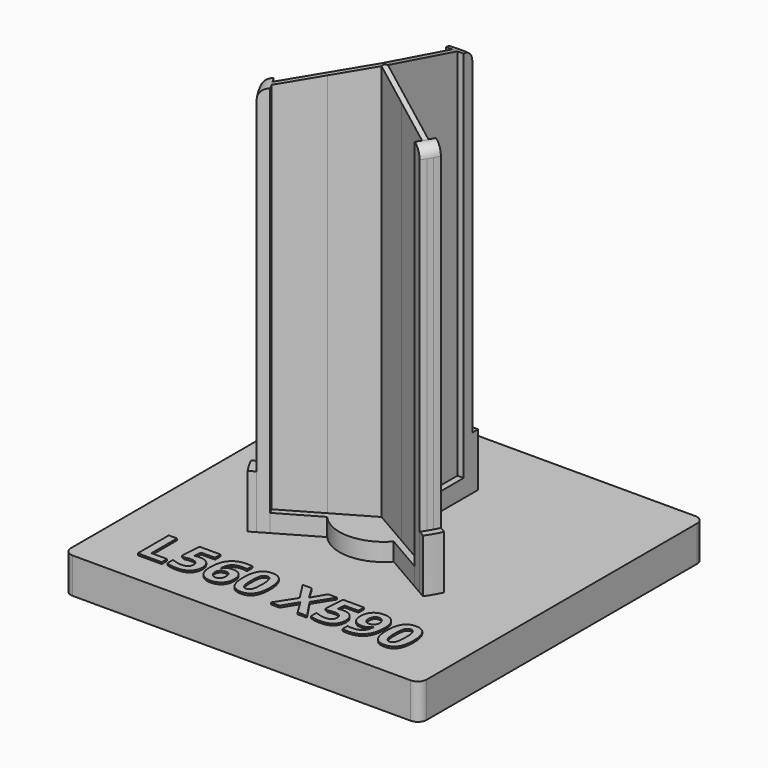
from build123d import *

# Parameters (mm, degrees)
F0_R         = 3.5
F0_R_2       = 1.75
F1_DEPTH     = 10
F2_DEPTH     = 220
F3_DEPTH     = 235
F4_T4_DEPTH  = 293.7329049929
F4_T9_DEPTH  = 293.7329049929
F4_T14_DEPTH = 293.7329049929
F5_T2_ANGLE  = 40.9393595263
F5_T4_ANGLE  = 40.9393595263
F5_T6_ANGLE  = 40.9393595263
F6_DEPTH     = 3
F7_DEPTH     = 30
F8_W         = 200
F8_H         = 200
F9_DEPTH     = 20
F10_R        = 5
F0_TEXT_SIZE = 30.5555555556
F11_DEPTH    = 1


# Not quite as in the source:
# - a fillet or chamfer that OpenCascade refuses, or shapes differently, is made with other operations: its cross-section is extruded or revolved along the edge and cut away or added
# - a feature names something its author has since deleted; it is built from what else it names
# - Text() gives the source's letters only with a copy of the font that has no kerning and outlines rounded to 1/6400 em; it was checked with that copy


with BuildPart() as f1:
    # F0 (on Top) → F1 (new body)
    with BuildSketch(Plane.XY):
        with BuildLine():
            ThreePointArc((25, 0), (19.364916731, 15.8113883008), (5, 24.4948974278))
            ThreePointArc((5, 24.4948974278), (3.2581304855, 24.7867824806), (1.5, 24.9549594269))
            Line((1.5, 24.9549594269), (1.5, 0.8660254038))
            Line((1.5, 0.8660254038), (22.3616288141, -11.1784416078))
            ThreePointArc((22.3616288141, -11.1784416078), (23.095048549, -9.571767471), (23.7132034356, -7.917321695))
            ThreePointArc((23.7132034356, -7.917321695), (24.6762039817, -4.0106055721), (25, 0))
        make_face()
        with Locations((11.9308144071, 6.8882589096)):
            Circle(F0_R, mode=Mode.SUBTRACT)
        with BuildLine():
            Line((5, 24.4948974278), (5, 49.7493718553))
            Line((5, 49.7493718553), (1.5, 49.7493718553))
            Line((1.5, 49.7493718553), (1.5, 24.9549594269))
            ThreePointArc((1.5, 24.9549594269), (3.2581304855, 24.7867824806), (5, 24.4948974278))
        make_face()
        with BuildLine():
            Line((43.834219849, -23.575647822), (45.584219849, -20.5445589087))
            Line((45.584219849, -20.5445589087), (23.7132034356, -7.917321695))
            ThreePointArc((23.7132034356, -7.917321695), (23.095048549, -9.571767471), (22.3616288141, -11.1784416078))
            Line((22.3616288141, -11.1784416078), (43.834219849, -23.575647822))
        make_face()
        with Locations((11.9308144071, 6.8882589096)):
            Circle(F0_R)
        with Locations((11.9308144071, 6.8882589096)):
            Circle(F0_R_2, mode=Mode.SUBTRACT)
        with Locations((11.9308144071, 6.8882589096)):
            Circle(F0_R_2)
    extrude(amount=F1_DEPTH)



with BuildPart() as f1b:
    # F0 (on Top) → F1, piece 2 (new body)
    with BuildSketch(Plane.XY):
        with BuildLine():
            Line((-1.5, 49.7493718553), (-5, 49.7493718553))
            Line((-5, 49.7493718553), (-5, 24.4948974278))
            ThreePointArc((-5, 24.4948974278), (-3.2581304855, 24.7867824806), (-1.5, 24.9549594269))
            Line((-1.5, 24.9549594269), (-1.5, 49.7493718553))
        make_face()
        with BuildLine():
            Line((-23.7132034356, -7.917321695), (-45.584219849, -20.5445589087))
            Line((-45.584219849, -20.5445589087), (-43.834219849, -23.575647822))
            Line((-43.834219849, -23.575647822), (-22.3616288141, -11.1784416078))
            ThreePointArc((-22.3616288141, -11.1784416078), (-23.095048549, -9.571767471), (-23.7132034356, -7.917321695))
        make_face()
        with BuildLine():
            ThreePointArc((-1.5, 24.9549594269), (-3.2581304855, 24.7867824806), (-5, 24.4948974278))
            ThreePointArc((-5, 24.4948974278), (-21.6506350946, 12.5), (-23.7132034356, -7.917321695))
            ThreePointArc((-23.7132034356, -7.917321695), (-23.095048549, -9.571767471), (-22.3616288141, -11.1784416078))
            Line((-22.3616288141, -11.1784416078), (-1.5, 0.8660254038))
            Line((-1.5, 0.8660254038), (-1.5, 24.9549594269))
        make_face()
        with Locations((-11.9308144071, 6.8882589096)):
            Circle(F0_R, mode=Mode.SUBTRACT)
        with Locations((-11.9308144071, 6.8882589096)):
            Circle(F0_R)
        with Locations((-11.9308144071, 6.8882589096)):
            Circle(F0_R_2, mode=Mode.SUBTRACT)
        with Locations((-11.9308144071, 6.8882589096)):
            Circle(F0_R_2)
    extrude(amount=F1_DEPTH)


with BuildPart() as f1c:
    # F0 (on Top) → F1, piece 3 (new body)
    with BuildSketch(Plane.XY):
        with BuildLine():
            ThreePointArc((-18.7132034356, -16.5775757328), (0, -25), (18.7132034356, -16.5775757328))
            ThreePointArc((18.7132034356, -16.5775757328), (19.8369180635, -15.2150150096), (20.8616288141, -13.7765178191))
            Line((20.8616288141, -13.7765178191), (0, -1.7320508076))
            Line((0, -1.7320508076), (-20.8616288141, -13.7765178191))
            ThreePointArc((-20.8616288141, -13.7765178191), (-19.8369180635, -15.2150150096), (-18.7132034356, -16.5775757328))
        make_face()
        with Locations((0, -13.7765178191)):
            Circle(F0_R, mode=Mode.SUBTRACT)
        with BuildLine():
            Line((18.7132034356, -16.5775757328), (40.584219849, -29.2048129466))
            Line((40.584219849, -29.2048129466), (42.334219849, -26.1737240333))
            Line((42.334219849, -26.1737240333), (20.8616288141, -13.7765178191))
            ThreePointArc((20.8616288141, -13.7765178191), (19.8369180635, -15.2150150096), (18.7132034356, -16.5775757328))
        make_face()
        with BuildLine():
            Line((-42.334219849, -26.1737240333), (-40.584219849, -29.2048129466))
            Line((-40.584219849, -29.2048129466), (-18.7132034356, -16.5775757328))
            ThreePointArc((-18.7132034356, -16.5775757328), (-19.8369180635, -15.2150150096), (-20.8616288141, -13.7765178191))
            Line((-20.8616288141, -13.7765178191), (-42.334219849, -26.1737240333))
        make_face()
        with Locations((0, -13.7765178191)):
            Circle(F0_R)
        with Locations((0, -13.7765178191)):
            Circle(F0_R_2, mode=Mode.SUBTRACT)
        with Locations((0, -13.7765178191)):
            Circle(F0_R_2)
    extrude(amount=F1_DEPTH)


with BuildPart() as f1_1:
    add(f1.part)

    add(f1b.part)  # F2 merges F1b

    add(f1c.part)  # F2 merges F1c
    # F0 (on Top) → F2 (join)
    with BuildSketch(Plane.XY):
        with BuildLine():
            Line((5, 49.7493718553), (5, 55.7763390695))
            ThreePointArc((5, 55.7763390695), (3.2515934535, 55.9055197634), (1.5, 55.9799071096))
            Line((1.5, 55.9799071096), (1.5, 49.7493718553))
            Line((1.5, 49.7493718553), (5, 49.7493718553))
        make_face()
        with BuildLine():
            ThreePointArc((-1.5, 55.9799071096), (-3.2515934535, 55.9055197634), (-5, 55.7763390695))
            Line((-5, 55.7763390695), (-5, 49.7493718553))
            Line((-5, 49.7493718553), (-1.5, 49.7493718553))
            Line((-1.5, 49.7493718553), (-1.5, 55.9799071096))
        make_face()
        with BuildLine():
            ThreePointArc((-47.7300216584, -29.2889916605), (-46.7898036001, -30.7687224152), (-45.8037265643, -32.2182965537))
            Line((-45.8037265643, -32.2182965537), (-40.584219849, -29.2048129466))
            Line((-40.584219849, -29.2048129466), (-42.334219849, -26.1737240333))
            Line((-42.334219849, -26.1737240333), (-47.7300216584, -29.2889916605))
        make_face()
        with BuildLine():
            Line((-45.584219849, -20.5445589087), (-50.8037265643, -23.5580425158))
            ThreePointArc((-50.8037265643, -23.5580425158), (-50.0413970536, -25.1367973482), (-49.2300216584, -26.6909154491))
            Line((-49.2300216584, -26.6909154491), (-43.834219849, -23.575647822))
            Line((-43.834219849, -23.575647822), (-45.584219849, -20.5445589087))
        make_face()
        with BuildLine():
            Line((40.584219849, -29.2048129466), (45.8037265643, -32.2182965537))
            ThreePointArc((45.8037265643, -32.2182965537), (46.7898036001, -30.7687224152), (47.7300216584, -29.2889916605))
            Line((47.7300216584, -29.2889916605), (42.334219849, -26.1737240333))
            Line((42.334219849, -26.1737240333), (40.584219849, -29.2048129466))
        make_face()
        with BuildLine():
            ThreePointArc((49.2300216584, -26.6909154491), (50.0413970536, -25.1367973482), (50.8037265643, -23.5580425158))
            Line((50.8037265643, -23.5580425158), (45.584219849, -20.5445589087))
            Line((45.584219849, -20.5445589087), (43.834219849, -23.575647822))
            Line((43.834219849, -23.575647822), (49.2300216584, -26.6909154491))
        make_face()
        with BuildLine():
            Line((-43.834219849, -23.575647822), (-49.2300216584, -26.6909154491))
            ThreePointArc((-49.2300216584, -26.6909154491), (-48.4974226119, -28), (-47.7300216584, -29.2889916605))
            Line((-47.7300216584, -29.2889916605), (-42.334219849, -26.1737240333))
            Line((-42.334219849, -26.1737240333), (-43.834219849, -23.575647822))
        make_face()
        with BuildLine():
            ThreePointArc((47.7300216584, -29.2889916605), (48.4974226119, -28), (49.2300216584, -26.6909154491))
            Line((49.2300216584, -26.6909154491), (43.834219849, -23.575647822))
            Line((43.834219849, -23.575647822), (42.334219849, -26.1737240333))
            Line((42.334219849, -26.1737240333), (47.7300216584, -29.2889916605))
        make_face()
        with BuildLine():
            Line((1.5, 49.7493718553), (1.5, 55.9799071096))
            ThreePointArc((1.5, 55.9799071096), (0, 56), (-1.5, 55.9799071096))
            Line((-1.5, 55.9799071096), (-1.5, 49.7493718553))
            Line((-1.5, 49.7493718553), (1.5, 49.7493718553))
        make_face()
    extrude(amount=F2_DEPTH)

    # F0 (on Top) → F3 (join)
    with BuildSketch(Plane.XY):
        with BuildLine():
            Line((1.5, 0.8660254038), (1.5, 24.9549594269))
            ThreePointArc((1.5, 24.9549594269), (0, 25), (-1.5, 24.9549594269))
            Line((-1.5, 24.9549594269), (-1.5, 0.8660254038))
            Line((-1.5, 0.8660254038), (-22.3616288141, -11.1784416078))
            ThreePointArc((-22.3616288141, -11.1784416078), (-21.6506350946, -12.5), (-20.8616288141, -13.7765178191))
            Line((-20.8616288141, -13.7765178191), (0, -1.7320508076))
            Line((0, -1.7320508076), (20.8616288141, -13.7765178191))
            ThreePointArc((20.8616288141, -13.7765178191), (21.6506350946, -12.5), (22.3616288141, -11.1784416078))
            Line((22.3616288141, -11.1784416078), (1.5, 0.8660254038))
        make_face()
        with BuildLine():
            Line((1.5, 24.9549594269), (1.5, 49.7493718553))
            Line((1.5, 49.7493718553), (-1.5, 49.7493718553))
            Line((-1.5, 49.7493718553), (-1.5, 24.9549594269))
            ThreePointArc((-1.5, 24.9549594269), (0, 25), (1.5, 24.9549594269))
        make_face()
        with BuildLine():
            Line((-22.3616288141, -11.1784416078), (-43.834219849, -23.575647822))
            Line((-43.834219849, -23.575647822), (-42.334219849, -26.1737240333))
            Line((-42.334219849, -26.1737240333), (-20.8616288141, -13.7765178191))
            ThreePointArc((-20.8616288141, -13.7765178191), (-21.6506350946, -12.5), (-22.3616288141, -11.1784416078))
        make_face()
        with BuildLine():
            Line((42.334219849, -26.1737240333), (43.834219849, -23.575647822))
            Line((43.834219849, -23.575647822), (22.3616288141, -11.1784416078))
            ThreePointArc((22.3616288141, -11.1784416078), (21.6506350946, -12.5), (20.8616288141, -13.7765178191))
            Line((20.8616288141, -13.7765178191), (42.334219849, -26.1737240333))
        make_face()
    extrude(amount=F3_DEPTH)

    # F4: chamfer of 15 x 55.9807621135 on 3 edges, made by hand


with BuildPart() as f4_tool2:
    # F4_s3 → F4_t4 (new body)
    with BuildSketch(Plane(origin=(-73.4332262482, -127.1900788256, 0), x_dir=(0, 0, 1), z_dir=(0.5, 0.8660254038, 0))):
        Polygon((220, 49.7493718553), (235, -6.2313902582), (235, 49.7493718553), align=None)
    extrude(amount=F4_T4_DEPTH)

    split(bisect_by=Plane.XY.offset(220), keep=Keep.TOP)


with BuildPart() as f1_2:
    add(f1_1.part)

    # F4_t1: cut F4_tool2
    add(f4_tool2.part, mode=Mode.SUBTRACT)


with BuildPart() as f4_tool7:
    # F4_s8 → F4_t9 (new body)
    with BuildSketch(Plane(origin=(-73.4332262482, 127.1900788256, 0), x_dir=(0, 0, 1), z_dir=(0.5, -0.8660254038, 0))):
        Polygon((235, -6.2313902582), (220, 49.7493718553), (235, 49.7493718553), align=None)
    extrude(amount=F4_T9_DEPTH)

    split(bisect_by=Plane.XY.offset(220), keep=Keep.TOP)


with BuildPart() as f1_3:
    add(f1_2.part)

    # F4_t6: cut F4_tool7
    add(f4_tool7.part, mode=Mode.SUBTRACT)


with BuildPart() as f4_tool12:
    # F4_s13 → F4_t14 (new body)
    with BuildSketch(Plane.YZ.offset(146.8664524965)):
        Polygon((-6.2313902582, 235), (49.7493718553, 220), (49.7493718553, 235), align=None)
    extrude(amount=-F4_T14_DEPTH)

    split(bisect_by=Plane.XY.offset(220), keep=Keep.TOP)


with BuildPart() as f1_4:
    add(f1_3.part)

    # F4_t11: cut F4_tool12
    add(f4_tool12.part, mode=Mode.SUBTRACT)

    # F5: fillet of radius 6 on 3 edges, made by hand

    # F5_s1 → F5_t2 (revolve, cut)
    with BuildSketch(Plane(origin=(0, 0, 0), x_dir=(0, 0, 1), z_dir=(-0.7712878704, -0.6364864656, 0))):
        with BuildLine():
            ThreePointArc((220, -50), (218.2426406871, -54.2426406871), (214, -56))
            Line((214, -56), (220, -56))
            Line((220, -56), (220, -50))
        make_face()
    revolve(axis=Axis((0, 0, 220), (0, 0, 1)), revolution_arc=F5_T2_ANGLE, mode=Mode.SUBTRACT)

    # F5_s3 → F5_t4 (revolve, cut)
    with BuildSketch(Plane(origin=(0, 0, 0), x_dir=(0, 0, 1), z_dir=(0.9368573836, -0.3497116566, 0))):
        with BuildLine():
            ThreePointArc((214, -56), (218.2426406871, -54.2426406871), (220, -50))
            Line((220, -50), (220, -56))
            Line((220, -56), (214, -56))
        make_face()
    revolve(axis=Axis((0, 0, 220), (0, 0, 1)), revolution_arc=F5_T4_ANGLE, mode=Mode.SUBTRACT)

    # F5_s5 → F5_t6 (revolve, cut)
    with BuildSketch(Plane(origin=(0, 0, 0), x_dir=(0, 0, 1), z_dir=(-0.1655695132, 0.9861981222, 0))):
        with BuildLine():
            ThreePointArc((214, -56), (218.2426406871, -54.2426406871), (220, -50))
            Line((220, -50), (220, -56))
            Line((220, -56), (214, -56))
        make_face()
    revolve(axis=Axis((0, 0, 220), (0, 0, 1)), revolution_arc=F5_T6_ANGLE, mode=Mode.SUBTRACT)

    # F0 (on Top) → F6 (join)
    with BuildSketch(Plane.XY):
        with Locations((-11.9308144071, 6.8882589096)):
            Circle(F0_R)
        with Locations((-11.9308144071, 6.8882589096)):
            Circle(F0_R_2, mode=Mode.SUBTRACT)
        with Locations((0, -13.7765178191)):
            Circle(F0_R)
        with Locations((0, -13.7765178191)):
            Circle(F0_R_2, mode=Mode.SUBTRACT)
        with Locations((11.9308144071, 6.8882589096)):
            Circle(F0_R)
        with Locations((11.9308144071, 6.8882589096)):
            Circle(F0_R_2, mode=Mode.SUBTRACT)
    extrude(amount=F6_DEPTH)

    # F0 (on Top) → F7 (join)
    with BuildSketch(Plane.XY):
        with BuildLine():
            Line((-50.8037265643, -23.5580425158), (-54.280787943, -25.5655248388))
            ThreePointArc((-54.280787943, -25.5655248388), (-51.9615242271, -30), (-49.280787943, -34.2257788767))
            Line((-49.280787943, -34.2257788767), (-45.8037265643, -32.2182965537))
            ThreePointArc((-45.8037265643, -32.2182965537), (-46.7898036001, -30.7687224152), (-47.7300216584, -29.2889916605))
            ThreePointArc((-47.7300216584, -29.2889916605), (-48.4974226119, -28), (-49.2300216584, -26.6909154491))
            ThreePointArc((-49.2300216584, -26.6909154491), (-50.0413970536, -25.1367973482), (-50.8037265643, -23.5580425158))
        make_face()
        with BuildLine():
            ThreePointArc((49.280787943, -34.2257788767), (51.9615242271, -30), (54.280787943, -25.5655248388))
            Line((54.280787943, -25.5655248388), (50.8037265643, -23.5580425158))
            ThreePointArc((50.8037265643, -23.5580425158), (50.0413970536, -25.1367973482), (49.2300216584, -26.6909154491))
            ThreePointArc((49.2300216584, -26.6909154491), (48.4974226119, -28), (47.7300216584, -29.2889916605))
            ThreePointArc((47.7300216584, -29.2889916605), (46.7898036001, -30.7687224152), (45.8037265643, -32.2182965537))
            Line((45.8037265643, -32.2182965537), (49.280787943, -34.2257788767))
        make_face()
        with BuildLine():
            Line((5, 55.7763390695), (5, 59.7913037155))
            ThreePointArc((5, 59.7913037155), (0, 60), (-5, 59.7913037155))
            Line((-5, 59.7913037155), (-5, 55.7763390695))
            ThreePointArc((-5, 55.7763390695), (-3.2515934535, 55.9055197634), (-1.5, 55.9799071096))
            ThreePointArc((-1.5, 55.9799071096), (0, 56), (1.5, 55.9799071096))
            ThreePointArc((1.5, 55.9799071096), (3.2515934535, 55.9055197634), (5, 55.7763390695))
        make_face()
    extrude(amount=F7_DEPTH)

    # F8 (on Top) → F9 (join)
    with BuildSketch(Plane.XY):
        Rectangle(F8_W, F8_H)
    extrude(amount=-F9_DEPTH)

    # F10
    f10_edges = [f1_4.edges().sort_by_distance(p)[0] for p in [
        (-100, -100, -10),
        (100, -100, -10),
        (100, 100, -10),
        (-100, 100, -10),
    ]]
    fillet(f10_edges, radius=F10_R)

    # F0 (on Top) → F11 (join)
    with BuildSketch(Plane.XY):
        with Locations((-75.560546875, -82)):
            Text('L560 X590', F0_TEXT_SIZE, font='Open Sans', font_style=FontStyle.BOLD, text_align=(TextAlign.LEFT, TextAlign.BOTTOM))
    extrude(amount=F11_DEPTH)


solid = f1_4.part
